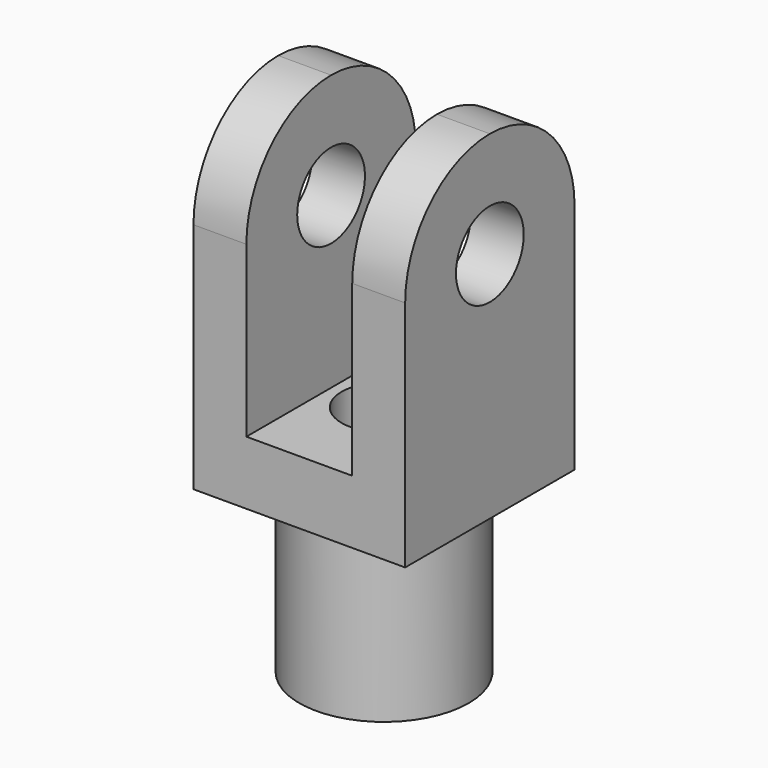
from build123d import *

# Parameters (mm, degrees)
F1_DEPTH = 50
F2_R     = 24.99999
F4_D     = 20
F5_R     = 20
F6_DEPTH = 40
F8_D     = 20


# Not quite as in the source:
# - a fillet or chamfer is up to 0.001 mm smaller than in the source, because OpenCascade refuses the exact size


with BuildPart() as f1:
    # F0 (on Front) → F1 (new body)
    with BuildSketch(Plane.XZ):
        Polygon((-25, 0), (0, 0), (25, 0), (25, 80), (12.5, 80), (12.5, 15), (0, 15), (-12.5, 15), (-12.5, 80), (-25, 80), align=None)
    extrude(amount=F1_DEPTH)

    # F2 (radius 25 in the source; OpenCascade refuses exactly that, so slightly less here)
    f2_edges = [f1.edges().sort_by_distance(p)[0] for p in [
        (18.75, 0, 80),
        (-18.75, 0, 80),
        (-18.75, -50, 80),
        (18.75, -50, 80),
    ]]
    fillet(f2_edges, radius=F2_R)

    # F4 (through all)
    with Locations(Plane.YZ.offset(25)):
        with Locations((-25, 55)):
            Hole(F4_D / 2)

    # F5 (on face) → F6 (join)
    with BuildSketch(Plane(origin=(0, 0, 0), x_dir=(1, 0, 0), z_dir=(0, 0, -1))):
        with Locations((0, 25)):
            Circle(F5_R)
    extrude(amount=F6_DEPTH)

    # F8 (through all)
    with Locations(Plane(origin=(0, 0, -40), x_dir=(1, 0, 0), z_dir=(0, 0, -1))):
        with Locations((0, 25)):
            Hole(F8_D / 2)


solid = f1.part
